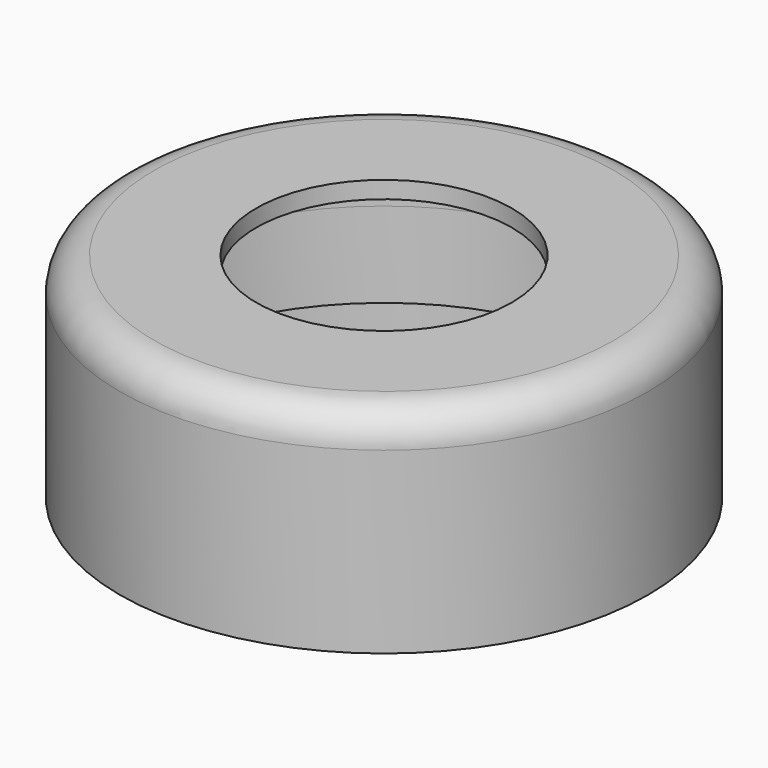
from build123d import *

# Parameters (mm, degrees)
F0_R      = 39.37
F1_DEPTH  = 12.7
F2_T      = -2.54
F3_R      = 5.08
F4_R      = 2.54
F5_R      = 19.05
F6_DEPTH  = 25.4
F7_R      = 39.37
F7_R_2    = 1.0414
F7_R_3    = 1.016
F8_DEPTH  = 12.7
F9_R      = 39.37
F9_R_2    = 38.1
F10_DEPTH = 6.35


with BuildPart() as f1:
    # F0 (on Top) → F1 (new body)
    with BuildSketch(Plane.XY):
        Circle(F0_R)
    extrude(amount=F1_DEPTH)

    # F2
    f2_openings = [f1.faces().sort_by_distance(p)[0] for p in [
        (0, 0, 0),
    ]]
    offset(amount=F2_T, openings=f2_openings)

    # F3
    f3_edges = [f1.edges().sort_by_distance(p)[0] for p in [
        (-39.37, 0, 12.7),
    ]]
    fillet(f3_edges, radius=F3_R)

    # F4
    f4_edges = [f1.edges().sort_by_distance(p)[0] for p in [
        (-36.83, 0, 10.16),
    ]]
    fillet(f4_edges, radius=F4_R)

    # F5 (on face) → F6 (cut)
    with BuildSketch(Plane(origin=(0, 0, 10.16), x_dir=(1, 0, 0), z_dir=(0, 0, -1))):
        Circle(F5_R)
    extrude(amount=-F6_DEPTH, mode=Mode.SUBTRACT)

    # F7 (on face) → F8 (join)
    with BuildSketch(Plane(origin=(0, 0, 0), x_dir=(1, 0, 0), z_dir=(0, 0, -1))):
        Circle(F7_R)
        with BuildLine():
            ThreePointArc((18.923, -31.5969772447), (-29.1572661412, -22.5011717733), (-25.7682217594, 26.3144))
            Line((-25.7682217594, 26.3144), (18.923, 26.3144))
            Line((18.923, 26.3144), (18.923, -31.5969772447))
        make_face(mode=Mode.SUBTRACT)
        with Locations((25.5778, -9.3218)):
            Circle(F7_R_2, mode=Mode.SUBTRACT)
        with Locations((0, 28.3972)):
            Circle(F7_R_3, mode=Mode.SUBTRACT)
    extrude(amount=F8_DEPTH)

    # F9 (on face) → F10 (join)
    with BuildSketch(Plane(origin=(0, 0, -12.7), x_dir=(1, 0, 0), z_dir=(0, 0, -1))):
        Circle(F9_R)
        Circle(F9_R_2, mode=Mode.SUBTRACT)
    extrude(amount=F10_DEPTH)


solid = f1.part
